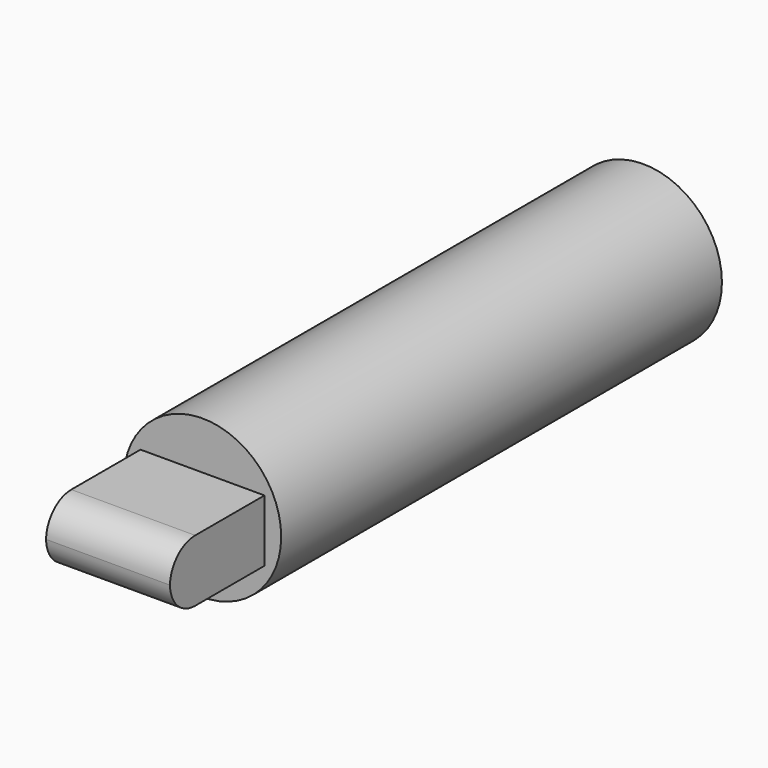
from build123d import *

# Parameters (mm, degrees)
F0_R        = 12.7
F1_DEPTH    = 88.9
F2_W        = 20
F2_H        = 10
F3_DEPTH    = 19.05
F4_T1_DEPTH = 45.4


# Not quite as in the source:
# - a fillet or chamfer that OpenCascade refuses, or shapes differently, is made with other operations: its cross-section is extruded or revolved along the edge and cut away or added


with BuildPart() as f1:
    # F0 (on Front) → F1 (new body)
    with BuildSketch(Plane.XZ):
        Circle(F0_R)
    extrude(amount=F1_DEPTH)

    # F2 (on face) → F3 (join)
    with BuildSketch(Plane.XZ.offset(88.9)):
        Rectangle(F2_W, F2_H)
    extrude(amount=F3_DEPTH)

    # F4: fillet of radius 5.08 on 2 edges, made by hand

    # F4_s2 → F4_t1 (cut)
    with BuildSketch(Plane.YZ.offset(-22.7)):
        with BuildLine():
            ThreePointArc((-102.87, 5), (-106.4621024484, 3.5121024484), (-107.95, -0.08))
            Line((-107.95, -0.08), (-107.95, 5))
            Line((-107.95, 5), (-102.87, 5))
        make_face()
        with BuildLine():
            ThreePointArc((-102.87, -5), (-106.4621024484, -3.5121024484), (-107.95, 0.08))
            Line((-107.95, 0.08), (-107.95, -5))
            Line((-107.95, -5), (-102.87, -5))
        make_face()
    extrude(amount=F4_T1_DEPTH, mode=Mode.SUBTRACT)


solid = f1.part
